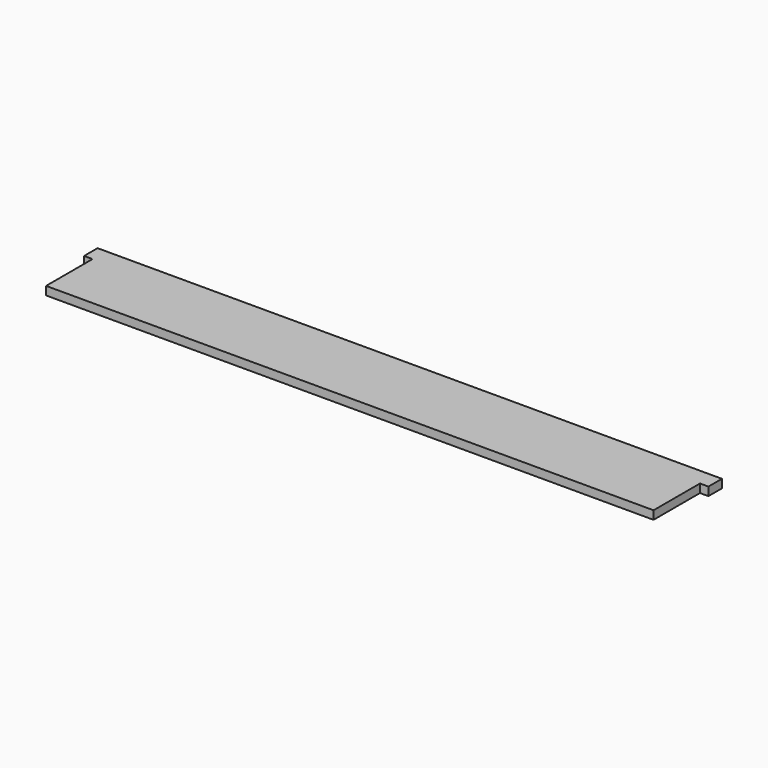
from build123d import *

# Parameters (mm, degrees)
F0_W     = 3.175
F0_H     = 6.35
F1_DEPTH = 3.175


# Not quite as in the source:
# - a length typed as a fraction of an inch, garbled in the dataset ("3 / 203.2 mm" for 3/8 in), is restored


with BuildPart() as f1:
    # F0 (on Top) → F1 (new body)
    with BuildSketch(Plane.XY):
        Polygon((228.6, 0), (0, 0), (0, -6.35), (0, -28.194), (228.6, -28.194), (228.6, -6.35), align=None)
        with Locations((230.1875, -3.175)):
            Rectangle(F0_W, F0_H)
        with Locations((-1.5875, -3.175)):
            Rectangle(F0_W, F0_H)
    extrude(amount=F1_DEPTH)


solid = f1.part
